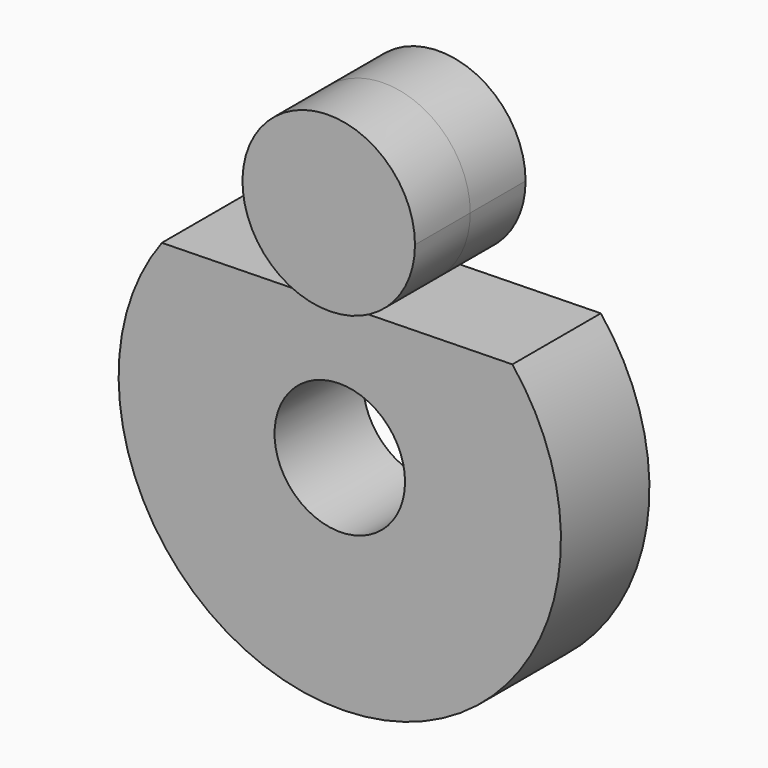
from build123d import *

# Parameters (mm, degrees)
F0_R     = 2.9972
F1_DEPTH = 2.54
F2_DEPTH = 3.175


# Not quite as in the source:
# - a feature names something its author has since deleted; it is built from what else it names


with BuildPart() as f1:
    # F0 (on Front) → F1 (new body, symmetric)
    with BuildSketch(Plane.XZ):
        with BuildLine():
            Line((0.078317611, 6.1990582674), (-8.172718603, 6.0359150621))
            ThreePointArc((-8.172718603, 6.0359150621), (0.2008488403, -10.1580145572), (7.9277344701, 6.354260474))
            Line((7.9277344701, 6.354260474), (0.078317611, 6.1990582674))
        make_face()
        Circle(F0_R, mode=Mode.SUBTRACT)
    extrude(amount=F1_DEPTH, both=True)


with BuildPart() as f2:
    # F0 (on Front) → F2 (new body, symmetric)
    with BuildSketch(Plane.XZ):
        with BuildLine():
            ThreePointArc((3.9617159233, 10.16), (-2.828910142, 12.9335285225), (0.078317611, 6.1990582674))
            ThreePointArc((0.078317611, 6.1990582674), (2.828910142, 7.3864714775), (3.9617159233, 10.16))
        make_face()
    extrude(amount=F2_DEPTH, both=True)


solid = Compound([f1.part, f2.part])
